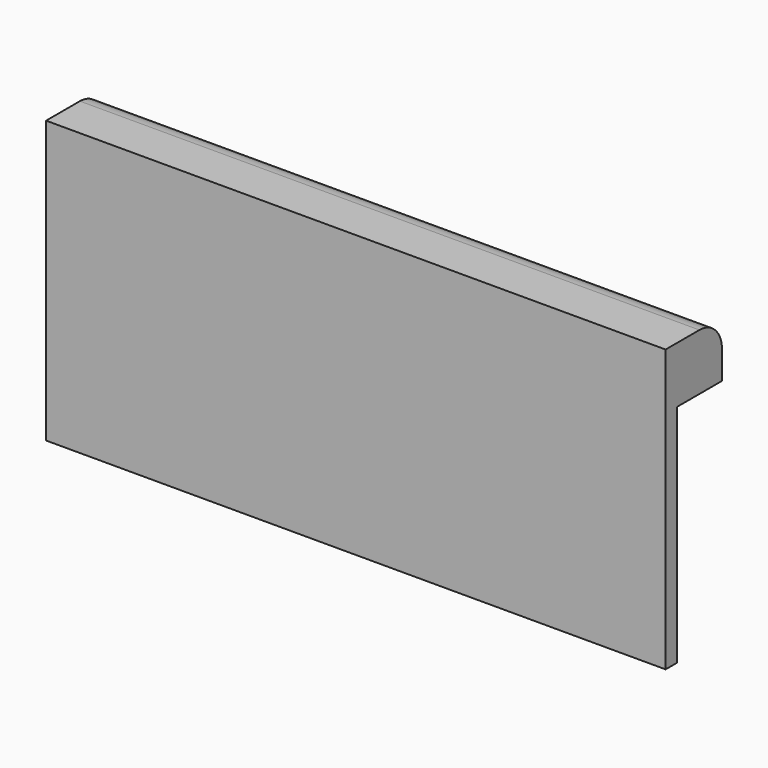
from build123d import *

# Parameters (mm, degrees)
F0_W     = 279.4
F0_H     = 101.6
F1_DEPTH = 6.35
F2_DEPTH = 25.4
F3_T     = -6.35
F4_R     = 12.7


# Not quite as in the source:
# - a shell that OpenCascade refuses in one call is made with other operations: the cavity is built on its own and cut out


with BuildPart() as f1:
    # F0 (on Front) → F1 (new body)
    with BuildSketch(Plane.XZ):
        with Locations((0, -12.7)):
            Rectangle(F0_W, F0_H)
        Polygon((-139.7, 38.1), (139.7, 38.1), (139.7, 50.8), (0, 50.8), (-139.7, 50.8), align=None)
        Polygon((0, 50.8), (139.7, 50.8), (139.7, 63.5), (-139.7, 63.5), (-139.7, 50.8), align=None)
    extrude(amount=F1_DEPTH)

    # F0 (on Front) → F2 (join)
    with BuildSketch(Plane.XZ):
        Polygon((0, 50.8), (139.7, 50.8), (139.7, 63.5), (-139.7, 63.5), (-139.7, 50.8), align=None)
        Polygon((-139.7, 38.1), (139.7, 38.1), (139.7, 50.8), (0, 50.8), (-139.7, 50.8), align=None)
    extrude(amount=-F2_DEPTH)

    # F3: a shell. OpenCascade refuses it in one call, so the cavity is built on its own and cut out:
    # the body offset inwards by the wall thickness, plus a prism from it out through each open face.
    f3_core = offset(f1.part, amount=F3_T, kind=Kind.INTERSECTION, mode=Mode.PRIVATE)
    f3_exits = [f3_core.faces().sort_by_distance(p)[0] for p in [
        (0, 9.525, 44.45),
    ]]
    add(f3_core, mode=Mode.SUBTRACT)
    extrude(f3_exits, amount=-F3_T, mode=Mode.SUBTRACT)

    # F4
    f4_edges = [f1.edges().sort_by_distance(p)[0] for p in [
        (0, 25.4, 63.5),
    ]]
    fillet(f4_edges, radius=F4_R)


solid = f1.part
